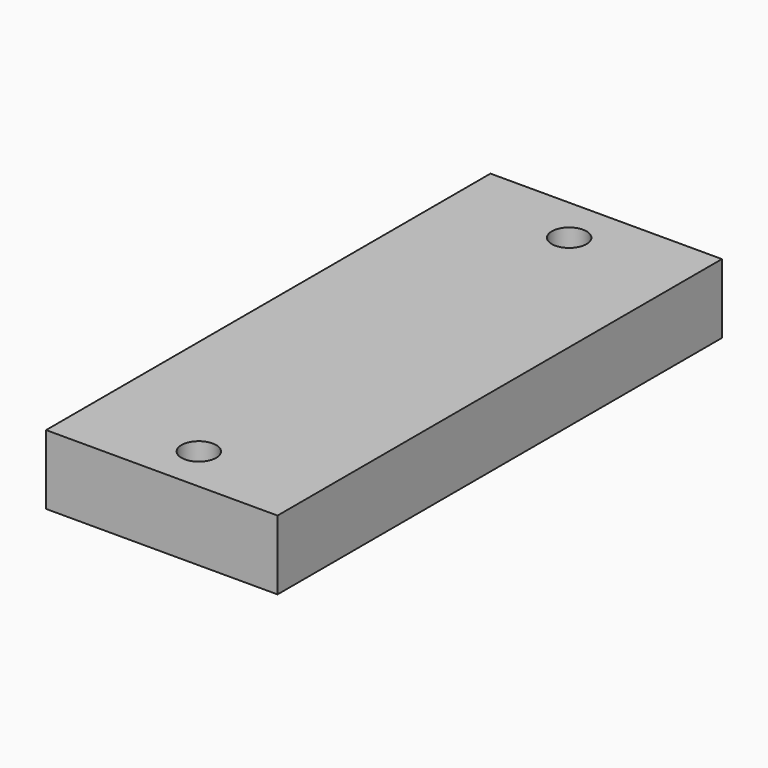
from build123d import *

# Parameters (mm, degrees)
F0_W     = 63.5
F0_H     = 152.4
F1_DEPTH = 19.05
F3_D     = 9.525
F3_DEPTH = 19.05
F3_TIP   = 2.8615986981


# Not quite as in the source:
# - a length typed as a fraction of an inch, garbled in the dataset ("3 / 203.2 mm" for 3/8 in), is restored


with BuildPart() as f1:
    # F0 (on Top) → F1 (new body)
    with BuildSketch(Plane.XY):
        Rectangle(F0_W, F0_H)
    extrude(amount=F1_DEPTH)

    # F3
    with Locations(Plane.XY.offset(19.05)):
        with Locations((0, -63.5), (0, 63.5)):
            Hole(F3_D / 2, depth=F3_DEPTH)
            with Locations((0, 0, -(F3_DEPTH + F3_TIP / 2))):  # 118° drill point
                Cone(0, F3_D / 2, F3_TIP, mode=Mode.SUBTRACT)


solid = f1.part
